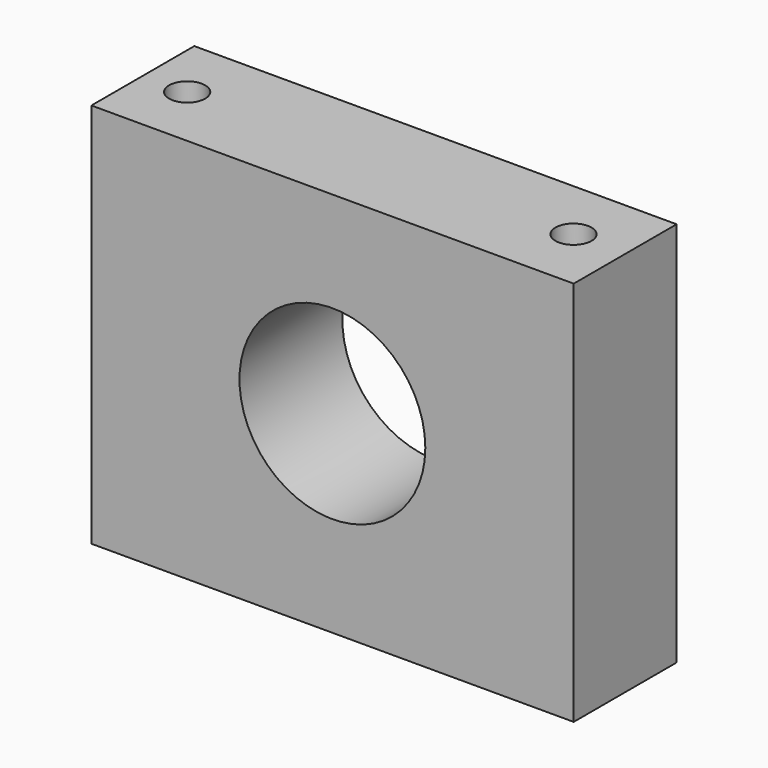
from build123d import *

# Parameters (mm, degrees)
F1_DEPTH = 25.4
F2_R     = 3.5687
F3_DEPTH = 7.1374
F4_DEPTH = 7.1374


# Not quite as in the source:
# - a feature names something its author has since deleted; it is built from what else it names


with BuildPart() as f1:
    # F0 (on Front) → F1 (new body)
    with BuildSketch(Plane.XZ):
        with BuildLine():
            Line((47.6553842176, 38.1), (-47.5946157824, 38.1))
            Line((-47.5946157824, 38.1), (-47.5946157824, 0))
            Line((-47.5946157824, 0), (-18.3505333031, 0))
            ThreePointArc((-18.3505333031, 0), (0, 18.3505333031), (18.3505333031, 0))
            Line((18.3505333031, 0), (47.6553842176, 0))
            Line((47.6553842176, 0), (47.6553842176, 38.1))
        make_face()
        with BuildLine():
            Line((-18.3505333031, 0), (-47.5946157824, 0))
            Line((-47.5946157824, 0), (-47.5946157824, -38.1))
            Line((-47.5946157824, -38.1), (47.6553842176, -38.1))
            Line((47.6553842176, -38.1), (47.6553842176, 0))
            Line((47.6553842176, 0), (18.3505333031, 0))
            ThreePointArc((18.3505333031, 0), (0, -18.3505333031), (-18.3505333031, 0))
        make_face()
    extrude(amount=F1_DEPTH)

    # F2 (on face) → F3 (cut)
    with BuildSketch(Plane.XY.offset(38.1)):
        with Locations((37.3155283745, -12.5269582962)):
            Circle(F2_R)
    extrude(amount=-F3_DEPTH, mode=Mode.SUBTRACT)

    # F2 (on face) → F4 (cut)
    with BuildSketch(Plane.XY.offset(38.1)):
        with Locations((-38.8844716255, -12.6503112141)):
            Circle(F2_R)
        with Locations((37.3155283745, -12.5269582962)):
            Circle(F2_R)
    extrude(amount=-F4_DEPTH, mode=Mode.SUBTRACT)


solid = f1.part
